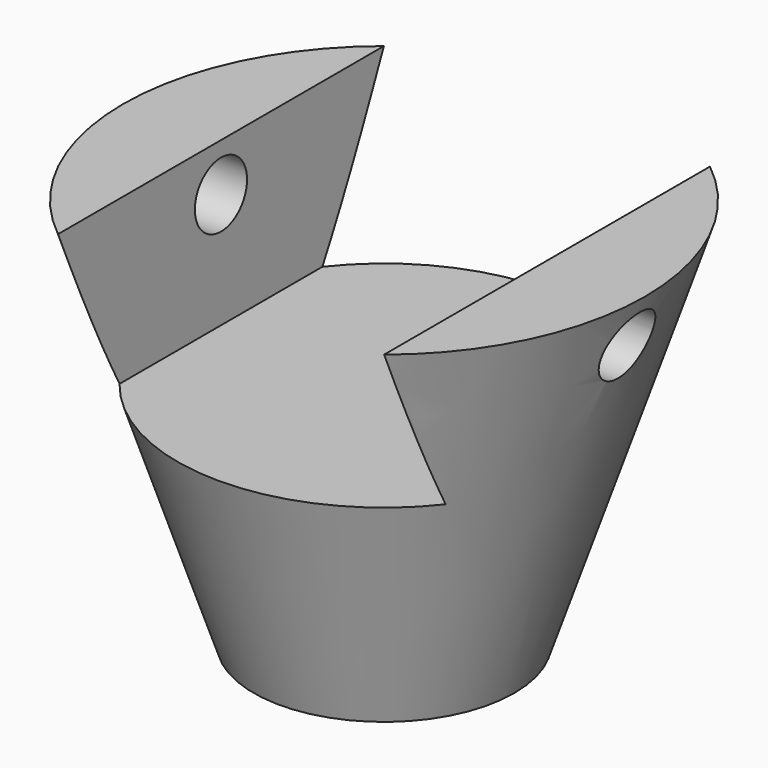
from build123d import *

# Parameters (mm, degrees)
F0_R     = 25.4
F2_R     = 50.8
F5_DEPTH = 31.75
F7_R     = 6.35
F8_DEPTH = 127


# Not quite as in the source:
# - a feature names something its author has since deleted; it is built from what else it names


with BuildPart() as f3:
    # F0 (on Top) → F3 section 0
    with BuildSketch(Plane.XY):
        Circle(F0_R)
    # F2 (on offset) → F3 section 1
    with BuildSketch(Plane.XY.offset(76.2)):
        Circle(F2_R)
    loft()

    # F4 (on face) → F5 (cut)
    with BuildSketch(Plane.XY.offset(76.2)):
        with BuildLine():
            Line((31.75, -39.6557372898), (31.75, 39.6557372898))
            ThreePointArc((31.75, 39.6557372898), (0, 50.8), (-31.75, 39.6557372898))
            Line((-31.75, 39.6557372898), (-31.75, -39.6557372898))
            ThreePointArc((-31.75, -39.6557372898), (0, -50.8), (31.75, -39.6557372898))
        make_face()
    extrude(amount=-F5_DEPTH, mode=Mode.SUBTRACT)

    # F7 (on offset) → F8 (cut)
    with BuildSketch(Plane.YZ.offset(50.8)):
        with Locations((0, 66.8615028262)):
            Circle(F7_R)
    extrude(amount=-F8_DEPTH, mode=Mode.SUBTRACT)


solid = f3.part
